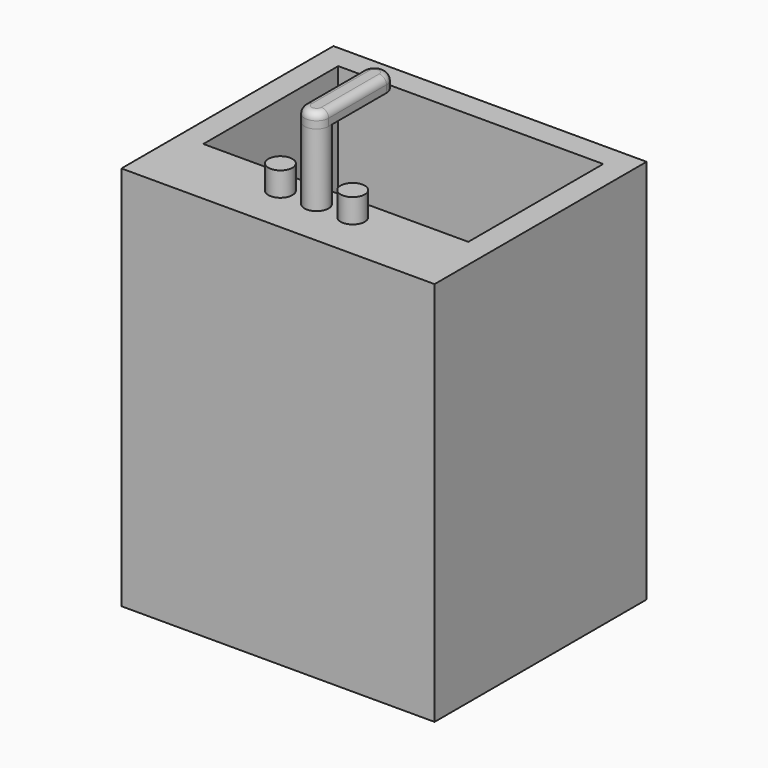
from build123d import *

# Parameters (mm, degrees)
F0_W     = 13
F0_H     = 11
F1_DEPTH = 16
F2_W     = 11
F2_H     = 7
F3_DEPTH = 6
F4_R     = 0.5
F5_R     = 0.5
F6_DEPTH = 1
F7_DEPTH = 3
F9_DEPTH = 0.6
F10_R    = 0.3


# Not quite as in the source:
# - a feature names something its author has since deleted; it is built from what else it names


with BuildPart() as f1:
    # F0 (on Top) → F1 (new body)
    with BuildSketch(Plane.XY):
        with Locations((6.5, 5.5)):
            Rectangle(F0_W, F0_H)
    extrude(amount=F1_DEPTH)

    # F2 (on face) → F3 (cut)
    with BuildSketch(Plane.XY.offset(16)):
        with Locations((6.5, 6.5)):
            Rectangle(F2_W, F2_H)
    extrude(amount=-F3_DEPTH, mode=Mode.SUBTRACT)

    # F4
    f4_edges = [f1.edges().sort_by_distance(p)[0] for p in [
        (1, 6.5, 10),
        (6.5, 3, 10),
        (12, 6.5, 10),
        (6.5, 10, 10),
    ]]
    fillet(f4_edges, radius=F4_R)

    # F5 (on face) → F6 (join)
    with BuildSketch(Plane.XY.offset(16)):
        with Locations((5, 2)):
            Circle(F5_R)
        with Locations((8, 2)):
            Circle(F5_R)
    extrude(amount=F6_DEPTH)

    # F5 (on face) → F7 (join)
    with BuildSketch(Plane.XY.offset(16)):
        with Locations((6.5, 2)):
            Circle(F5_R)
    extrude(amount=F7_DEPTH)

    # F8 (on face) → F9 (join)
    with BuildSketch(Plane.XY.offset(19)):
        with BuildLine():
            Line((6, 5), (6, 2))
            ThreePointArc((6, 2), (6.5, 1.5), (7, 2))
            Line((7, 2), (7, 5))
            ThreePointArc((7, 5), (6.5, 5.5), (6, 5))
        make_face()
    extrude(amount=F9_DEPTH)

    # F10
    f10_edges = [f1.edges().sort_by_distance(p)[0] for p in [
        (6, 3.5, 19.6),
        (6.5, 1.5, 19.6),
        (7, 3.5, 19.6),
        (6.5, 5.5, 19.6),
    ]]
    fillet(f10_edges, radius=F10_R)


solid = f1.part
